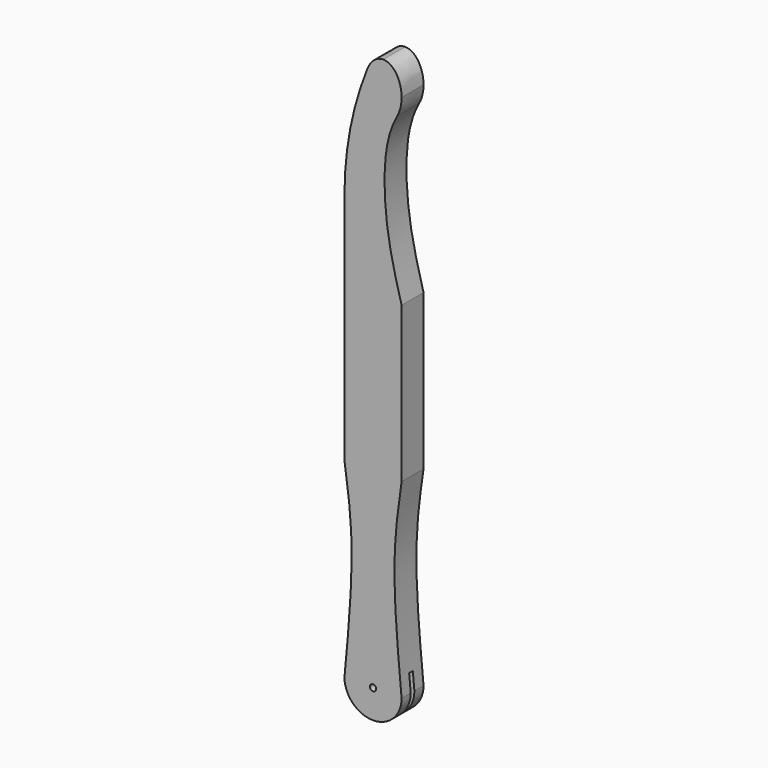
from build123d import *

# Parameters (mm, degrees)
F0_W     = 39.6875
F0_H     = 406.4
F1_DEPTH = 9.525
F2_W     = 6.35
F2_H     = 39.6875
F3_DEPTH = 25
F5_DEPTH = 19.051
F7_DEPTH = 1.5875
F9_D     = 4.318


with BuildPart() as f1:
    # F0 (on Front) → F1 (new body, symmetric)
    with BuildSketch(Plane.XZ):
        Rectangle(F0_W, F0_H)
    extrude(amount=F1_DEPTH, both=True)

    # F2 (on face) → F3 (cut)
    with BuildSketch(Plane(origin=(-19.84375, 0, 0), x_dir=(0, -1, 0), z_dir=(-1, 0, 0))):
        Rectangle(F2_W, F2_H)
    extrude(amount=-F3_DEPTH, mode=Mode.SUBTRACT)

    # F4 (on face) → F5 (cut, through all)
    with BuildSketch(Plane.XZ.offset(9.525)):
        with BuildLine():
            Line((7.0341385432, 203.2), (-19.84375, 203.2))
            Line((-19.84375, 203.2), (-19.84375, 111.521875))
            ThreePointArc((-19.84375, 111.521875), (-15.8400316853, 153.4647609056), (-3.9734854925, 193.8927279568))
            add(Edge.make_bspline(
                [(7.0341385432, 203.2), (-0.2487850546, 203.2), (-3.9734854925, 193.8927279568)],
                knots=[0, 0, 0, 1.0339490894, 1.0339490894, 1.0339490894], degree=2, weights=[1, 0.8693184943, 1]))
        make_face()
        with BuildLine():
            Line((19.84375, 203.2), (7.0341385432, 203.2))
            add(Edge.make_bspline(
                [(19.84375, 184.1499997199), (19.8437501883, 203.2), (7.0341385432, 203.2)],
                knots=[4.7123889657, 4.7123889657, 4.7123889657, 6.2831853072, 6.2831853072, 6.2831853072], degree=2, weights=[1, 0.707106776, 1]))
            Line((19.84375, 184.1499997199), (19.84375, 203.2))
        make_face()
        with BuildLine():
            Line((19.84375, 176.5695613803), (19.84375, 184.1499997199))
            add(Edge.make_bspline(
                [(16.84439979, 171.9005189458), (19.8437499314, 177.2131309179), (19.84375, 184.1499997199)],
                knots=[4.0139573004, 4.0139573004, 4.0139573004, 4.7123889657, 4.7123889657, 4.7123889657], degree=2, weights=[1, 0.9396413133, 1]))
            add(Edge.make_bspline(
                [(19.84375, 176.5695613803), (18.8065478073, 175.1509160959), (17.8010548966, 173.5949984606), (16.84439979, 171.9005189458)],
                knots=[0, 0, 0, 0, 0.0662671427, 0.0662671427, 0.0662671427, 0.0662671427], degree=3))
        make_face()
        with BuildLine():
            add(Edge.make_bspline(
                [(19.84375, 176.5695613803), (18.8065478073, 175.1509160959), (17.8010548966, 173.5949984606), (16.84439979, 171.9005189458)],
                knots=[0, 0, 0, 0, 0.0662671427, 0.0662671427, 0.0662671427, 0.0662671427], degree=3))
            add(Edge.make_bspline(
                [(16.84439979, 171.9005189458), (13.9150462786, 166.7118888088), (6.871998352, 148.2229851045), (7.9533512774, 100.8460076909), (16.1750007742, 70.447095167), (19.84375, 57.1321291334)],
                knots=[0.0662671427, 0.0662671427, 0.0662671427, 0.0662671427, 0.2691823685, 0.6445312257, 1, 1, 1, 1], degree=3))
            Line((19.84375, 57.1321291334), (19.84375, 176.5695613803))
        make_face()
        with BuildLine():
            add(Edge.make_bspline(
                [(-19.84375, -50.8), (-17.5374013822, -66.7231403213), (-12.3094439018, -102.8172091965), (-17.1427124069, -154.4831051715), (-19.84375, -183.35625)],
                knots=[0, 0, 0, 0, 0.4411567231, 1, 1, 1, 1], degree=3))
            Line((-19.84375, -50.8), (-19.84375, -183.35625))
        make_face()
        with BuildLine():
            ThreePointArc((0, -203.2), (-14.0316501892, -197.3879001892), (-19.84375, -183.35625))
            Line((-19.84375, -183.35625), (-19.84375, -203.2))
            Line((-19.84375, -203.2), (0, -203.2))
        make_face()
        with BuildLine():
            Line((19.84375, -183.35625), (19.84375, -50.8))
            add(Edge.make_bspline(
                [(19.84375, -50.8), (17.5374013822, -66.7231403213), (12.3094439018, -102.8172091965), (17.1427124069, -154.4831051715), (19.84375, -183.35625)],
                knots=[0, 0, 0, 0, 0.4411567231, 1, 1, 1, 1], degree=3))
        make_face()
        with BuildLine():
            ThreePointArc((19.84375, -183.35625), (14.0316501892, -197.3879001892), (0, -203.2))
            Line((0, -203.2), (19.84375, -203.2))
            Line((19.84375, -203.2), (19.84375, -183.35625))
        make_face()
    extrude(amount=-F5_DEPTH, mode=Mode.SUBTRACT)

    # F6 (on Front) → F7 (cut, symmetric)
    with BuildSketch(Plane.XZ):
        with BuildLine():
            Line((15.875, -171.45), (-15.875, -171.45))
            ThreePointArc((-15.875, -171.45), (-18.8254341957, -177.0811052681), (-19.84375, -183.35625))
            ThreePointArc((-19.84375, -183.35625), (-14.0316501892, -197.3879001892), (0, -203.2))
            ThreePointArc((0, -203.2), (14.0316501892, -197.3879001892), (19.84375, -183.35625))
            ThreePointArc((19.84375, -183.35625), (18.8254341957, -177.0811052681), (15.875, -171.45))
        make_face()
        with BuildLine():
            ThreePointArc((-19.84375, -183.35625), (-18.8254341957, -177.0811052681), (-15.875, -171.45))
            Line((-15.875, -171.45), (-19.84375, -171.45))
            Line((-19.84375, -171.45), (-19.84375, -183.35625))
        make_face()
        with BuildLine():
            ThreePointArc((0, -203.2), (-14.0316501892, -197.3879001892), (-19.84375, -183.35625))
            Line((-19.84375, -183.35625), (-19.84375, -203.2))
            Line((-19.84375, -203.2), (0, -203.2))
        make_face()
        with BuildLine():
            Line((19.84375, -171.45), (15.875, -171.45))
            ThreePointArc((15.875, -171.45), (18.8254341957, -177.0811052681), (19.84375, -183.35625))
            Line((19.84375, -183.35625), (19.84375, -171.45))
        make_face()
        with BuildLine():
            ThreePointArc((19.84375, -183.35625), (14.0316501892, -197.3879001892), (0, -203.2))
            Line((0, -203.2), (19.84375, -203.2))
            Line((19.84375, -203.2), (19.84375, -183.35625))
        make_face()
    extrude(amount=F7_DEPTH, both=True, mode=Mode.SUBTRACT)

    # F9 (through all)
    with Locations(Plane.XZ.offset(9.525)):
        with Locations((0, -183.35625)):
            Hole(F9_D / 2)


solid = f1.part
